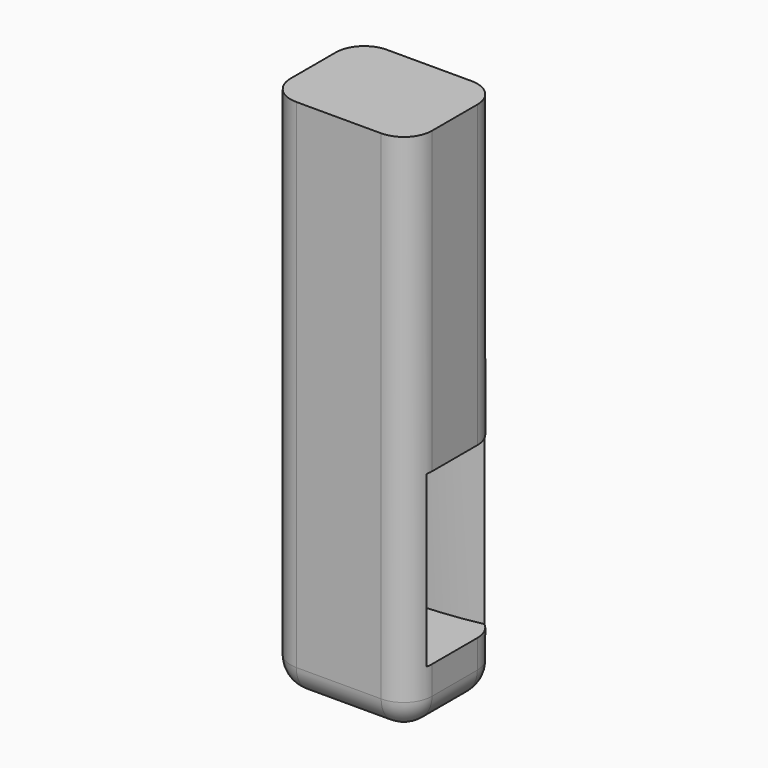
from build123d import *

# Parameters (mm, degrees)
F0_W         = 25
F0_H         = 20
F1_DEPTH     = 93
F3_R         = 80
F3_R_2       = 65
F4_DEPTH     = 30
F6_T1_DEPTH  = 10
F6_T3_DEPTH  = 15
F6_T5_DEPTH  = 100.5
F6_S9_W      = 5
F6_S9_H      = 5
F6_T10_DEPTH = 5
F6_S15_W     = 5
F6_S15_H     = 5
F6_T16_DEPTH = 5
F6_S21_W     = 5
F6_S21_H     = 5
F6_T22_DEPTH = 5
F6_S27_W     = 5
F6_S27_H     = 5
F6_T28_DEPTH = 5


# Not quite as in the source:
# - a fillet or chamfer that OpenCascade refuses, or shapes differently, is made with other operations: its cross-section is extruded or revolved along the edge and cut away or added


with BuildPart() as f1:
    # F0 (on Top) → F1 (new body)
    with BuildSketch(Plane.XY):
        with Locations((12.5, 0)):
            Rectangle(F0_W, F0_H)
    extrude(amount=F1_DEPTH)


with BuildPart() as f4:
    # F3 (on offset) → F4 (new body)
    with BuildSketch(Plane.XY.offset(10)):
        with Locations((10.065856821, 72.5)):
            Circle(F3_R)
        with Locations((10.065856821, 72.5)):
            Circle(F3_R_2, mode=Mode.SUBTRACT)
    extrude(amount=F4_DEPTH)


with BuildPart() as f1_1:
    add(f1.part)

    # F5: cut F4
    add(f4.part, mode=Mode.SUBTRACT)

    # F6: fillet of radius 5 on 8 edges, made by hand

    # F6_s2 → F6_t1 (cut)
    with BuildSketch(Plane.XZ.offset(-5)):
        with BuildLine():
            ThreePointArc((0, 5), (1.4644660941, 1.4644660941), (5, 0))
            Line((5, 0), (0, 0))
            Line((0, 0), (0, 5))
        make_face()
        with BuildLine():
            ThreePointArc((25, 5), (23.5355339059, 1.4644660941), (20, 0))
            Line((20, 0), (25, 0))
            Line((25, 0), (25, 5))
        make_face()
    extrude(amount=F6_T1_DEPTH, mode=Mode.SUBTRACT)

    # F6_s4 → F6_t3 (cut)
    with BuildSketch(Plane.YZ.offset(5)):
        with BuildLine():
            ThreePointArc((10, 5), (8.5355339059, 1.4644660941), (5, 0))
            Line((5, 0), (10, 0))
            Line((10, 0), (10, 5))
        make_face()
        with BuildLine():
            ThreePointArc((-5, 0), (-8.5355339059, 1.4644660941), (-10, 5))
            Line((-10, 5), (-10, 0))
            Line((-10, 0), (-5, 0))
        make_face()
    extrude(amount=F6_T3_DEPTH, mode=Mode.SUBTRACT)

    # F6_s6 → F6_t5 (cut)
    with BuildSketch(Plane.XY.offset(5)):
        with BuildLine():
            ThreePointArc((25, -5), (23.5355339059, -8.5355339059), (20, -10))
            Line((20, -10), (25, -10))
            Line((25, -10), (25, -5))
        make_face()
        with BuildLine():
            ThreePointArc((0, -5), (1.4644660941, -8.5355339059), (5, -10))
            Line((5, -10), (0, -10))
            Line((0, -10), (0, -5))
        make_face()
        with BuildLine():
            ThreePointArc((5, 10), (1.4644660941, 8.5355339059), (0, 5))
            Line((0, 5), (0, 10))
            Line((0, 10), (5, 10))
        make_face()
        with BuildLine():
            ThreePointArc((20, 10), (23.5355339059, 8.5355339059), (25, 5))
            Line((25, 5), (25, 10))
            Line((25, 10), (20, 10))
        make_face()
    extrude(amount=F6_T5_DEPTH, mode=Mode.SUBTRACT)


with BuildPart() as f6_tool8:
    # F6_s9 → F6_t10 (new body)
    with BuildSketch(Plane.XZ.offset(-5)):
        with Locations((2.5, 2.5)):
            Rectangle(F6_S9_W, F6_S9_H)
    extrude(amount=-F6_T10_DEPTH)

    # F6_s11 → F6_t12 (revolve, cut)
    with BuildSketch(Plane(origin=(5, 5, 5), x_dir=(0.7071067812, 0, 0.7071067812), z_dir=(-0.7071067812, 0, 0.7071067812))):
        with BuildLine():
            ThreePointArc((0, -5), (5, 0), (0, 5))
            Line((0, 5), (0, -5))
        make_face()
    revolve(axis=Axis((5, 5, 5), (0, 1, 0)), mode=Mode.SUBTRACT)


with BuildPart() as f1_2:
    add(f1_1.part)

    # F6_t7: cut F6_tool8
    add(f6_tool8.part, mode=Mode.SUBTRACT)


with BuildPart() as f6_tool14:
    # F6_s15 → F6_t16 (new body)
    with BuildSketch(Plane.YZ.offset(5)):
        with Locations((-7.5, 2.5)):
            Rectangle(F6_S15_W, F6_S15_H)
    extrude(amount=-F6_T16_DEPTH)

    # F6_s17 → F6_t18 (revolve, cut)
    with BuildSketch(Plane(origin=(5, -5, 5), x_dir=(0, 0.7071067812, 0.7071067812), z_dir=(0, -0.7071067812, 0.7071067812))):
        with BuildLine():
            ThreePointArc((0, -5), (5, 0), (0, 5))
            Line((0, 5), (0, -5))
        make_face()
    revolve(axis=Axis((5, -5, 5), (-1, 0, 0)), mode=Mode.SUBTRACT)


with BuildPart() as f1_3:
    add(f1_2.part)

    # F6_t13: cut F6_tool14
    add(f6_tool14.part, mode=Mode.SUBTRACT)


with BuildPart() as f6_tool20:
    # F6_s21 → F6_t22 (new body)
    with BuildSketch(Plane.XZ.offset(-5)):
        with Locations((22.5, 2.5)):
            Rectangle(F6_S21_W, F6_S21_H)
    extrude(amount=-F6_T22_DEPTH)

    # F6_s23 → F6_t24 (revolve, cut)
    with BuildSketch(Plane(origin=(20, 5, 5), x_dir=(-0.7071067812, 0, 0.7071067812), z_dir=(-0.7071067812, 0, -0.7071067812))):
        with BuildLine():
            ThreePointArc((0, -5), (5, 0), (0, 5))
            Line((0, 5), (0, -5))
        make_face()
    revolve(axis=Axis((20, 5, 5), (0, 1, 0)), mode=Mode.SUBTRACT)


with BuildPart() as f1_4:
    add(f1_3.part)

    # F6_t19: cut F6_tool20
    add(f6_tool20.part, mode=Mode.SUBTRACT)


with BuildPart() as f6_tool26:
    # F6_s27 → F6_t28 (new body)
    with BuildSketch(Plane.YZ.offset(20)):
        with Locations((-7.5, 2.5)):
            Rectangle(F6_S27_W, F6_S27_H)
    extrude(amount=F6_T28_DEPTH)

    # F6_s29 → F6_t30 (revolve, cut)
    with BuildSketch(Plane(origin=(20, -5, 5), x_dir=(0, 0.7071067812, 0.7071067812), z_dir=(0, 0.7071067812, -0.7071067812))):
        with BuildLine():
            ThreePointArc((0, -5), (5, 0), (0, 5))
            Line((0, 5), (0, -5))
        make_face()
    revolve(axis=Axis((20, -5, 5), (1, 0, 0)), mode=Mode.SUBTRACT)


with BuildPart() as f1_5:
    add(f1_4.part)

    # F6_t25: cut F6_tool26
    add(f6_tool26.part, mode=Mode.SUBTRACT)


solid = f1_5.part
